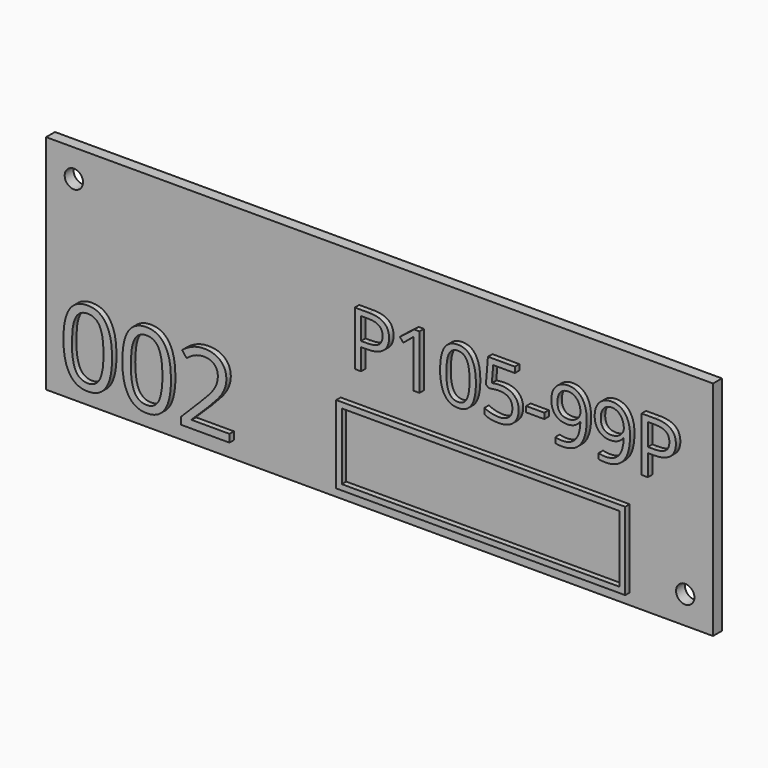
from build123d import *

# Parameters (mm, degrees)
F0_W         = 120
F0_H         = 40
F1_DEPTH     = 2
F3_D         = 3.3
F4_TEXT_SIZE = 13.6426617401
F5_DEPTH     = 1
F6_TEXT_SIZE = 18.5356140827
F7_DEPTH     = 1
F8_W         = 52
F8_H         = 14
F8_W_2       = 49.99999962
F8_H_2       = 11.99999962
F9_DEPTH     = 1


# Not quite as in the source:
# - Text() gives the source's letters only with a copy of the font that has no kerning and outlines rounded to 1/6400 em; it was checked with that copy


with BuildPart() as f1:
    # F0 (on Front) → F1 (new body)
    with BuildSketch(Plane.XZ):
        Rectangle(F0_W, F0_H)
    extrude(amount=F1_DEPTH)

    # F3 (through all)
    with Locations(Plane.XZ.offset(2)):
        with Locations((-55, 15), (55, -15)):
            Hole(F3_D / 2)

    # F4 (on face) → F5 (join)
    with BuildSketch(Plane.XZ.offset(2)):
        with Locations((-5, 2)):
            Text('P105-99P', F4_TEXT_SIZE, font='Open Sans', text_align=(TextAlign.LEFT, TextAlign.BOTTOM))
    extrude(amount=F5_DEPTH)

    # F6 (on face) → F7 (join)
    with BuildSketch(Plane.XZ.offset(2)):
        with Locations((-57, -17)):
            Text('002', F6_TEXT_SIZE, font='Open Sans', text_align=(TextAlign.LEFT, TextAlign.BOTTOM))
    extrude(amount=F7_DEPTH)

    # F8 (on face) → F9 (join)
    with BuildSketch(Plane.XZ.offset(2)):
        with Locations((19, -11)):
            Rectangle(F8_W, F8_H)
        with Locations((19, -11)):
            Rectangle(F8_W_2, F8_H_2, mode=Mode.SUBTRACT)
    extrude(amount=F9_DEPTH)


solid = f1.part
